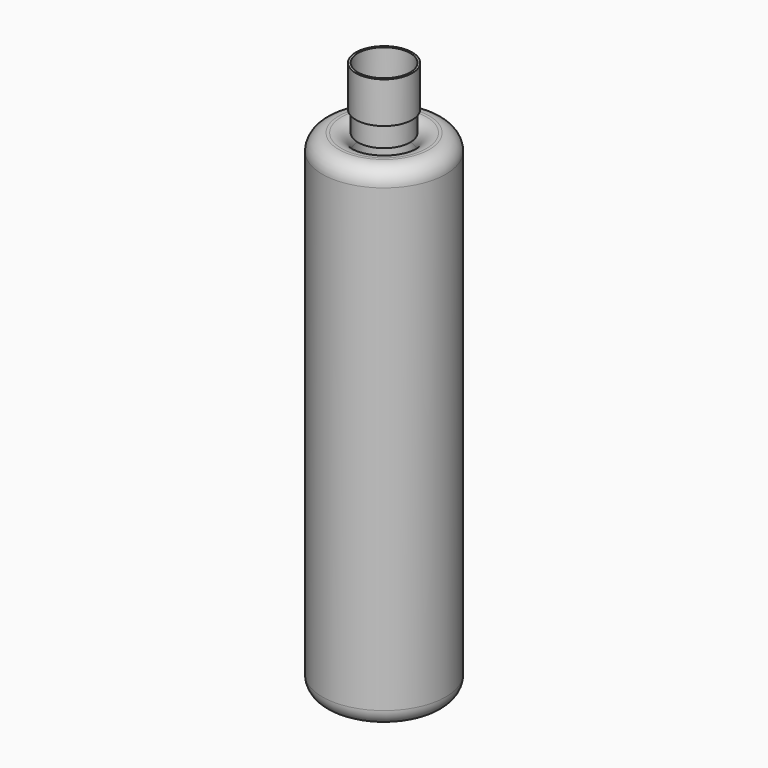
from build123d import *

# Parameters (mm, degrees)
F0_R     = 19.1010102766
F0_R_2   = 8.0791616643
F1_DEPTH = 76.2
F3_R     = 5.08
F2_R     = 8.0791616643
F4_DEPTH = 6.35
F6_R     = 5.08
F7_R     = 8.7181621078
F7_R_2   = 8.0791616643
F8_DEPTH = 12.7


with BuildPart() as f1:
    # F0 (on Top) → F1 (new body, symmetric)
    with BuildSketch(Plane.XY):
        Circle(F0_R)
        Circle(F0_R_2, mode=Mode.SUBTRACT)
    extrude(amount=F1_DEPTH, both=True)

    # F3
    f3_edges = [f1.edges().sort_by_distance(p)[0] for p in [
        (-19.10101, 0, -76.2),
    ]]
    fillet(f3_edges, radius=F3_R)

    # F6
    f6_edges = [f1.edges().sort_by_distance(p)[0] for p in [
        (-19.10101, 0, 76.2),
        (-8.079162, 0, 76.2),
    ]]
    fillet(f6_edges, radius=F6_R)


with BuildPart() as f4:
    # F2 (on face) → F4 (new body)
    with BuildSketch(Plane.XY.offset(76.2)):
        Circle(F2_R)
    extrude(amount=F4_DEPTH)


with BuildPart() as f8:
    # F7 (on face) → F8 (new body)
    with BuildSketch(Plane.XY.offset(82.55)):
        Circle(F7_R)
        Circle(F7_R_2, mode=Mode.SUBTRACT)
    extrude(amount=F8_DEPTH)


solid = Compound([f1.part, f4.part, f8.part])
